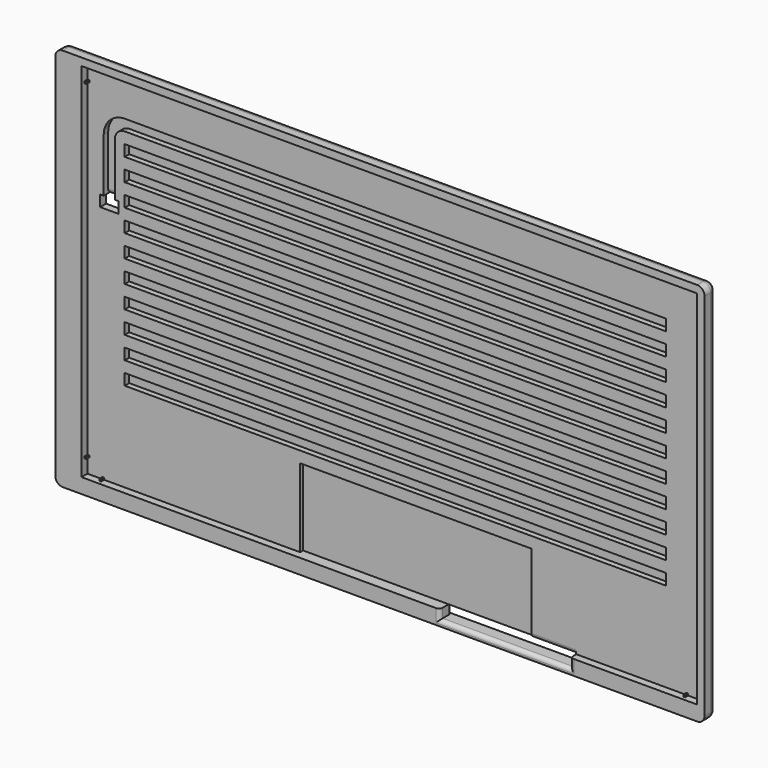
from build123d import *

# Parameters (mm, degrees)
F1_DEPTH     = 1
F0_W         = 145
F0_H         = 3
F2_DEPTH     = 2
F3_DEPTH     = 0.5
F0_W_2       = 0.5
F0_H_2       = 0.5
F4_DEPTH     = 3
F5_DEPTH     = 4
F6_T1_DEPTH  = 99
F6_T3_DEPTH  = 170
F6_T6_ANGLE  = 90
F6_T8_ANGLE  = 90
F6_T10_ANGLE = 90
F6_T12_ANGLE = 90
F7_T1_DEPTH  = 35
F7_T3_DEPTH  = 5
F7_T5_DEPTH  = 14.5
F7_T7_DEPTH  = 2.9999986291
F7_T12_DEPTH = 4.5
F7_T17_DEPTH = 4.5
F7_T23_DEPTH = 5
F7_T28_DEPTH = 37.5
F7_T35_DEPTH = 5
F7_T40_DEPTH = 37.5
F7_T47_DEPTH = 37.5
F7_T51_DEPTH = 7
F7_T58_DEPTH = 37.5
F7_T62_DEPTH = 7


# Not quite as in the source:
# - a fillet or chamfer that OpenCascade refuses, or shapes differently, is made with other operations: its cross-section is extruded or revolved along the edge and cut away or added
# - two fillets or chamfers of one size are made in one step
# - ends of sketch curves that miss each other by under 0.0002 mm in the source are joined
# - a feature names something its author has since deleted; it is built from what else it names


with BuildPart() as f1:
    # F0 (on Front) → F1 (new body)
    with BuildSketch(Plane.XZ):
        Polygon((-25.5, -27.5), (-25.5, -48.5), (13.5, -48.5), (36.5, -48.5), (36.5, -27.5), align=None)
    extrude(amount=F1_DEPTH)

    # F0 (on Front) → F2 (join)
    with BuildSketch(Plane.XZ):
        Polygon((-78.5, 48.5), (-82.5, 48.5), (-82.5, 44.5), (-82, 44.5), (-82, 44), (-82.5, 44), (-82.5, -44), (-82, -44), (-82, -44.5), (-82.5, -44.5), (-82.5, -48.5), (-78.5, -48.5), (-78.5, -48), (-78, -48), (-78, -48.5), (-25.5, -48.5), (-25.5, -27.5), (36.5, -27.5), (36.5, -48.5), (48.5, -48.5), (78, -48.5), (78, -48), (78.5, -48), (78.5, -48.5), (82.5, -48.5), (82.5, -44.5), (82, -44.5), (82, -44), (82.5, -44), (82.5, 44), (82, 44), (82, 44.5), (82.5, 44.5), (82.5, 48.5), (78.5, 48.5), (78.5, 48), (78, 48), (78, 48.5), (-78, 48.5), (-78, 48), (-78.5, 48), align=None)
        with Locations((0, -23)):
            Rectangle(F0_W, F0_H, mode=Mode.SUBTRACT)
        with Locations((0, -17)):
            Rectangle(F0_W, F0_H, mode=Mode.SUBTRACT)
        with Locations((0, -11)):
            Rectangle(F0_W, F0_H, mode=Mode.SUBTRACT)
        with Locations((0, -5)):
            Rectangle(F0_W, F0_H, mode=Mode.SUBTRACT)
        with BuildLine():
            ThreePointArc((-78.1382620335, 32.8617365956), (-76.486853318, 36.8485899136), (-72.5, 38.4999986291))
            Line((-72.5, 38.4999986291), (72.5, 38.5))
            Line((72.5, 38.5), (72.5, 35.5))
            Line((72.5, 35.5), (-72.5, 35.5))
            ThreePointArc((-72.5, 35.5), (-74.3655339438, 34.7272705394), (-75.1382634044, 32.8617365956))
            Line((-75.1382634044, 32.8617365956), (-75.1382634044, 18.5))
            Line((-75.1382634044, 18.5), (-74.2, 18.5))
            Line((-74.2, 18.5), (-74.2, 15.5))
            Line((-74.2, 15.5), (-79.1, 15.5))
            Line((-79.1, 15.5), (-79.1, 18.5))
            Line((-79.1, 18.5), (-78.1382620335, 18.5))
            Line((-78.1382620335, 18.5), (-78.1382620335, 32.8617365956))
        make_face(mode=Mode.SUBTRACT)
        with Locations((0, 1)):
            Rectangle(F0_W, F0_H, mode=Mode.SUBTRACT)
        with Locations((0, 7)):
            Rectangle(F0_W, F0_H, mode=Mode.SUBTRACT)
        with Locations((0, 13)):
            Rectangle(F0_W, F0_H, mode=Mode.SUBTRACT)
        with Locations((0, 19)):
            Rectangle(F0_W, F0_H, mode=Mode.SUBTRACT)
        with Locations((0, 25)):
            Rectangle(F0_W, F0_H, mode=Mode.SUBTRACT)
        with Locations((0, 31)):
            Rectangle(F0_W, F0_H, mode=Mode.SUBTRACT)
    extrude(amount=F2_DEPTH)

    # F0 (on Front) → F3 (join)
    with BuildSketch(Plane.XZ):
        with Locations((0, 37)):
            Rectangle(F0_W, F0_H)
        with Locations((0, 31)):
            Rectangle(F0_W, F0_H)
        with Locations((0, 25)):
            Rectangle(F0_W, F0_H)
        with Locations((0, 19)):
            Rectangle(F0_W, F0_H)
        with Locations((0, 13)):
            Rectangle(F0_W, F0_H)
        with Locations((0, 7)):
            Rectangle(F0_W, F0_H)
        with Locations((0, 1)):
            Rectangle(F0_W, F0_H)
        with Locations((0, -5)):
            Rectangle(F0_W, F0_H)
        with Locations((0, -11)):
            Rectangle(F0_W, F0_H)
        with Locations((0, -17)):
            Rectangle(F0_W, F0_H)
        with Locations((0, -23)):
            Rectangle(F0_W, F0_H)
        with BuildLine():
            Line((-72.5, 35.5), (-72.5, 38.5))
            ThreePointArc((-72.5, 38.5), (-76.486853318, 36.8485899136), (-78.1382620335, 32.8617365956))
            Line((-78.1382620335, 32.8617365956), (-78.1382620335, 18.5))
            Line((-78.1382620335, 18.5), (-75.1382634044, 18.5))
            Line((-75.1382634044, 18.5), (-75.1382634044, 32.8617365956))
            ThreePointArc((-75.1382634044, 32.8617365956), (-74.3655339438, 34.7272705394), (-72.5, 35.5))
        make_face()
    extrude(amount=F3_DEPTH)

    # F0 (on Front) → F4 (join)
    with BuildSketch(Plane.XZ):
        with Locations((-82.25, 44.25)):
            Rectangle(F0_W_2, F0_H_2)
        with Locations((-78.25, 48.25)):
            Rectangle(F0_W_2, F0_H_2)
        with Locations((-82.25, -44.25)):
            Rectangle(F0_W_2, F0_H_2)
        with Locations((-78.25, -48.25)):
            Rectangle(F0_W_2, F0_H_2)
        with Locations((82.25, -44.25)):
            Rectangle(F0_W_2, F0_H_2)
        with Locations((78.25, -48.25)):
            Rectangle(F0_W_2, F0_H_2)
        with Locations((78.25, 48.25)):
            Rectangle(F0_W_2, F0_H_2)
        with Locations((82.25, 44.25)):
            Rectangle(F0_W_2, F0_H_2)
    extrude(amount=F4_DEPTH)

    # F0 (on Front) → F5 (join)
    with BuildSketch(Plane.XZ):
        with BuildLine():
            Line((82.5, 50.5), (-87.5, 50.5))
            ThreePointArc((-87.5, 50.5), (-88.9142135624, 49.9142135624), (-89.5, 48.5))
            Line((-89.5, 48.5), (-89.5, -50.5))
            ThreePointArc((-89.5, -50.5), (-88.9142135624, -51.9142135624), (-87.5, -52.5))
            Line((-87.5, -52.5), (82.5, -52.5))
            ThreePointArc((82.5, -52.5), (83.9142135624, -51.9142135624), (84.5, -50.5))
            Line((84.5, -50.5), (84.5, 48.5))
            ThreePointArc((84.5, 48.5), (83.9142135624, 49.9142135624), (82.5, 50.5))
        make_face()
        Polygon((-82.5, 44.5), (-82.5, 48.5), (-78.5, 48.5), (-78, 48.5), (78, 48.5), (78.5, 48.5), (82.5, 48.5), (82.5, 44.5), (82.5, 44), (82.5, -44), (82.5, -44.5), (82.5, -48.5), (78.5, -48.5), (78, -48.5), (48.5, -48.5), (48.5, -51), (13.5, -51), (13.5, -48.5), (-25.5, -48.5), (-78, -48.5), (-78.5, -48.5), (-82.5, -48.5), (-82.5, -44.5), (-82.5, -44), (-82.5, 44), align=None, mode=Mode.SUBTRACT)
    extrude(amount=F5_DEPTH)

    # F6: fillet of radius 2 on 8 edges, made by hand

    # F6_s2 → F6_t1 (cut)
    with BuildSketch(Plane.XY.offset(-50.5)):
        with BuildLine():
            ThreePointArc((82.5, 0), (83.9142135624, -0.5857864376), (84.5, -2))
            Line((84.5, -2), (84.5, 0))
            Line((84.5, 0), (82.5, 0))
        make_face()
        with BuildLine():
            ThreePointArc((-87.5, 0), (-88.9142135624, -0.5857864376), (-89.5, -2))
            Line((-89.5, -2), (-89.5, 0))
            Line((-89.5, 0), (-87.5, 0))
        make_face()
    extrude(amount=F6_T1_DEPTH, mode=Mode.SUBTRACT)

    # F6_s4 → F6_t3 (cut)
    with BuildSketch(Plane.YZ.offset(-87.5)):
        with BuildLine():
            ThreePointArc((0, 48.5), (-0.5857864376, 49.9142135624), (-2, 50.5))
            Line((-2, 50.5), (0, 50.5))
            Line((0, 50.5), (0, 48.5))
        make_face()
        with BuildLine():
            ThreePointArc((0, -50.5), (-0.5857864376, -51.9142135624), (-2, -52.5))
            Line((-2, -52.5), (0, -52.5))
            Line((0, -52.5), (0, -50.5))
        make_face()
    extrude(amount=F6_T3_DEPTH, mode=Mode.SUBTRACT)

    # F6_s5 → F6_t6 (revolve, cut)
    with BuildSketch(Plane.YZ.offset(-87.5)):
        with BuildLine():
            ThreePointArc((0, 48.5), (-0.5857864376, 49.9142135624), (-2, 50.5))
            Line((-2, 50.5), (0, 50.5))
            Line((0, 50.5), (0, 48.5))
        make_face()
    revolve(axis=Axis((-87.5, 0, 48.5), (0, -1, 0)), revolution_arc=F6_T6_ANGLE, mode=Mode.SUBTRACT)

    # F6_s7 → F6_t8 (revolve, cut)
    with BuildSketch(Plane.XY.offset(-50.5)):
        with BuildLine():
            ThreePointArc((-87.5, 0), (-88.9142135624, -0.5857864376), (-89.5, -2))
            Line((-89.5, -2), (-89.5, 0))
            Line((-89.5, 0), (-87.5, 0))
        make_face()
    revolve(axis=Axis((-87.5, 0, -50.5), (0, -1, 0)), revolution_arc=F6_T8_ANGLE, mode=Mode.SUBTRACT)

    # F6_s9 → F6_t10 (revolve, cut)
    with BuildSketch(Plane.YZ.offset(82.5)):
        with BuildLine():
            ThreePointArc((0, -50.5), (-0.5857864376, -51.9142135624), (-2, -52.5))
            Line((-2, -52.5), (0, -52.5))
            Line((0, -52.5), (0, -50.5))
        make_face()
    revolve(axis=Axis((82.5, 0, -50.5), (0, -1, 0)), revolution_arc=F6_T10_ANGLE, mode=Mode.SUBTRACT)

    # F6_s11 → F6_t12 (revolve, cut)
    with BuildSketch(Plane.XY.offset(48.5)):
        with BuildLine():
            ThreePointArc((82.5, 0), (83.9142135624, -0.5857864376), (84.5, -2))
            Line((84.5, -2), (84.5, 0))
            Line((84.5, 0), (82.5, 0))
        make_face()
    revolve(axis=Axis((82.5, 0, 48.5), (0, -1, 0)), revolution_arc=F6_T12_ANGLE, mode=Mode.SUBTRACT)

    # F7: fillet of radius 1 on 8 edges, made by hand

    # F7_s2 → F7_t1 (cut)
    with BuildSketch(Plane.YZ.offset(13.5)):
        with BuildLine():
            ThreePointArc((-4, -52), (-3.7071067812, -51.2928932188), (-3, -51))
            Line((-3, -51), (-4, -51))
            Line((-4, -51), (-4, -52))
        make_face()
        with BuildLine():
            ThreePointArc((-1, -48.5), (-0.2928932188, -48.2071067812), (0, -47.5))
            Line((0, -47.5), (0, -48.5))
            Line((0, -48.5), (-1, -48.5))
        make_face()
    extrude(amount=F7_T1_DEPTH, mode=Mode.SUBTRACT)

    # F7_s4 → F7_t3 (cut)
    with BuildSketch(Plane.XY.offset(-51)):
        with BuildLine():
            ThreePointArc((48.5, -3), (48.7928932188, -3.7071067812), (49.5, -4))
            Line((49.5, -4), (48.5, -4))
            Line((48.5, -4), (48.5, -3))
        make_face()
        with BuildLine():
            ThreePointArc((13.5, -3), (13.2071067812, -3.7071067812), (12.5, -4))
            Line((12.5, -4), (13.5, -4))
            Line((13.5, -4), (13.5, -3))
        make_face()
    extrude(amount=F7_T3_DEPTH, mode=Mode.SUBTRACT)

    # F7_s6 → F7_t5 (cut)
    with BuildSketch(Plane.YZ.offset(34)):
        with BuildLine():
            ThreePointArc((-1, -48.5), (-1.7071067812, -48.2071067812), (-2, -47.5))
            Line((-2, -47.5), (-2, -48.5))
            Line((-2, -48.5), (-1, -48.5))
        make_face()
    extrude(amount=F7_T5_DEPTH, mode=Mode.SUBTRACT)

    # F7_s8 → F7_t7 (cut)
    with BuildSketch(Plane.YZ.offset(-78.1382620335)):
        with BuildLine():
            ThreePointArc((0.5, 18.5), (-0.2071067812, 18.7928932188), (-0.5, 19.5))
            Line((-0.5, 19.5), (-0.5, 18.5))
            Line((-0.5, 18.5), (0.5, 18.5))
        make_face()
    extrude(amount=F7_T7_DEPTH, mode=Mode.SUBTRACT)


with BuildPart() as f7_tool10:
    # F7_s11 → F7_t12 (new body)
    with BuildSketch(Plane.XY.offset(-53)):
        with BuildLine():
            ThreePointArc((13.5, -1), (13.2071067812, -0.2928932188), (12.5, 0))
            Line((12.5, 0), (13.5, 0))
            Line((13.5, 0), (13.5, -1))
        make_face()
    extrude(amount=F7_T12_DEPTH)

    split(bisect_by=Plane.XY.offset(-51), keep=Keep.TOP)


with BuildPart() as f1_1:
    add(f1.part)

    # F7_t9: cut F7_tool10
    add(f7_tool10.part, mode=Mode.SUBTRACT)


with BuildPart() as f7_tool15:
    # F7_s16 → F7_t17 (new body)
    with BuildSketch(Plane.XY.offset(-48.5)):
        with BuildLine():
            ThreePointArc((49.5, 0), (48.7928932188, -0.2928932188), (48.5, -1))
            Line((48.5, -1), (48.5, 0))
            Line((48.5, 0), (49.5, 0))
        make_face()
    extrude(amount=-F7_T17_DEPTH)

    split(bisect_by=Plane.XY.offset(-51), keep=Keep.TOP)


with BuildPart() as f1_2:
    add(f1_1.part)

    # F7_t14: cut F7_tool15
    add(f7_tool15.part, mode=Mode.SUBTRACT)


with BuildPart() as f7_tool21:
    # F7_s22 → F7_t23 (new body)
    with BuildSketch(Plane.XY.offset(-48.5)):
        with BuildLine():
            ThreePointArc((48.5, -3), (48.7928932188, -3.7071067812), (49.5, -4))
            Line((49.5, -4), (48.5, -4))
            Line((48.5, -4), (48.5, -3))
        make_face()
    extrude(amount=-F7_T23_DEPTH)

    split(bisect_by=Plane.XY.offset(-51), keep=Keep.BOTTOM)

    split(bisect_by=Plane.XY.offset(-52.5), keep=Keep.TOP)


with BuildPart() as f7_tool26:
    # F7_s27 → F7_t28 (new body)
    with BuildSketch(Plane.YZ.offset(51)):
        with BuildLine():
            ThreePointArc((-4, -52), (-3.7071067812, -51.2928932188), (-3, -51))
            Line((-3, -51), (-4, -51))
            Line((-4, -51), (-4, -52))
        make_face()
    extrude(amount=-F7_T28_DEPTH)

    split(bisect_by=Plane.YZ.offset(48.5), keep=Keep.TOP)


with BuildPart() as f7_tool21_1:
    add(f7_tool21.part)

    # F7_t30: intersect F7_tool26
    add(f7_tool26.part, mode=Mode.INTERSECT)


with BuildPart() as f1_3:
    add(f1_2.part)

    # F7_t19: cut F7_tool21
    add(f7_tool21_1.part, mode=Mode.SUBTRACT)


with BuildPart() as f7_tool33:
    # F7_s34 → F7_t35 (new body)
    with BuildSketch(Plane.XY.offset(-53.5)):
        with BuildLine():
            ThreePointArc((13.5, -3), (13.2071067812, -3.7071067812), (12.5, -4))
            Line((12.5, -4), (13.5, -4))
            Line((13.5, -4), (13.5, -3))
        make_face()
    extrude(amount=F7_T35_DEPTH)

    split(bisect_by=Plane.XY.offset(-51), keep=Keep.BOTTOM)

    split(bisect_by=Plane.XY.offset(-52.5), keep=Keep.TOP)


with BuildPart() as f7_tool38:
    # F7_s39 → F7_t40 (new body)
    with BuildSketch(Plane.YZ.offset(48.5)):
        with BuildLine():
            ThreePointArc((-4, -52), (-3.7071067812, -51.2928932188), (-3, -51))
            Line((-3, -51), (-4, -51))
            Line((-4, -51), (-4, -52))
        make_face()
    extrude(amount=-F7_T40_DEPTH)

    split(bisect_by=Plane.YZ.offset(13.5), keep=Keep.BOTTOM)


with BuildPart() as f7_tool33_1:
    add(f7_tool33.part)

    # F7_t42: intersect F7_tool38
    add(f7_tool38.part, mode=Mode.INTERSECT)


with BuildPart() as f1_4:
    add(f1_3.part)

    # F7_t31: cut F7_tool33
    add(f7_tool33_1.part, mode=Mode.SUBTRACT)


with BuildPart() as f7_tool45:
    # F7_s46 → F7_t47 (new body)
    with BuildSketch(Plane.YZ.offset(11)):
        with BuildLine():
            ThreePointArc((-1, -48.5), (-0.2928932188, -48.2071067812), (0, -47.5))
            Line((0, -47.5), (0, -48.5))
            Line((0, -48.5), (-1, -48.5))
        make_face()
    extrude(amount=F7_T47_DEPTH)

    split(bisect_by=Plane.YZ.offset(13.5), keep=Keep.BOTTOM)


with BuildPart() as f7_tool49:
    # F7_s50 → F7_t51 (new body)
    with BuildSketch(Plane.XY.offset(-53)):
        with BuildLine():
            ThreePointArc((13.5, -1), (13.2071067812, -0.2928932188), (12.5, 0))
            Line((12.5, 0), (13.5, 0))
            Line((13.5, 0), (13.5, -1))
        make_face()
    extrude(amount=F7_T51_DEPTH)

    split(bisect_by=Plane.XY.offset(-48.5), keep=Keep.TOP)


with BuildPart() as f7_tool45_1:
    add(f7_tool45.part)

    # F7_t53: intersect F7_tool49
    add(f7_tool49.part, mode=Mode.INTERSECT)


with BuildPart() as f1_5:
    add(f1_4.part)

    # F7_t43: cut F7_tool45
    add(f7_tool45_1.part, mode=Mode.SUBTRACT)


with BuildPart() as f7_tool56:
    # F7_s57 → F7_t58 (new body)
    with BuildSketch(Plane.YZ.offset(13.5)):
        with BuildLine():
            ThreePointArc((-1, -48.5), (-0.2928932188, -48.2071067812), (0, -47.5))
            Line((0, -47.5), (0, -48.5))
            Line((0, -48.5), (-1, -48.5))
        make_face()
    extrude(amount=F7_T58_DEPTH)

    split(bisect_by=Plane.YZ.offset(48.5), keep=Keep.TOP)


with BuildPart() as f7_tool60:
    # F7_s61 → F7_t62 (new body)
    with BuildSketch(Plane.XY.offset(-46)):
        with BuildLine():
            ThreePointArc((49.5, 0), (48.7928932188, -0.2928932188), (48.5, -1))
            Line((48.5, -1), (48.5, 0))
            Line((48.5, 0), (49.5, 0))
        make_face()
    extrude(amount=-F7_T62_DEPTH)

    split(bisect_by=Plane.XY.offset(-48.5), keep=Keep.TOP)


with BuildPart() as f7_tool56_1:
    add(f7_tool56.part)

    # F7_t64: intersect F7_tool60
    add(f7_tool60.part, mode=Mode.INTERSECT)


with BuildPart() as f1_6:
    add(f1_5.part)

    # F7_t54: cut F7_tool56
    add(f7_tool56_1.part, mode=Mode.SUBTRACT)


solid = f1_6.part
